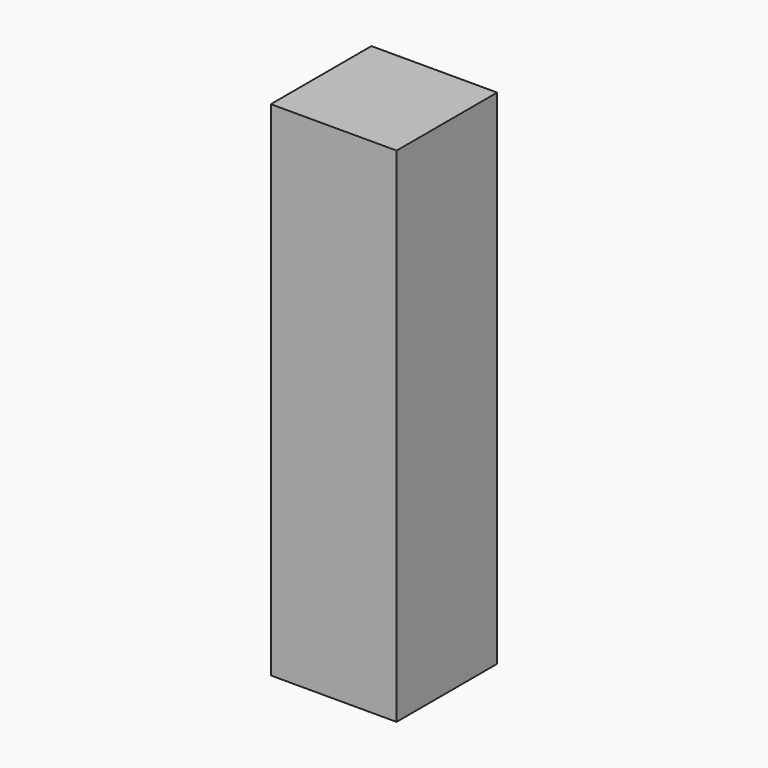
from build123d import *

# Parameters (mm, degrees)
F0_W     = 25.4
F0_H     = 101.6
F1_DEPTH = 25.4


# Not quite as in the source:
# - a feature names something its author has since deleted; it is built from what else it names


with BuildPart() as f1:
    # F0 (on Front) → F1 (new body)
    with BuildSketch(Plane.XZ):
        with Locations((-12.7, 3.8364605537)):
            Rectangle(F0_W, F0_H)
    extrude(amount=F1_DEPTH)


solid = f1.part
